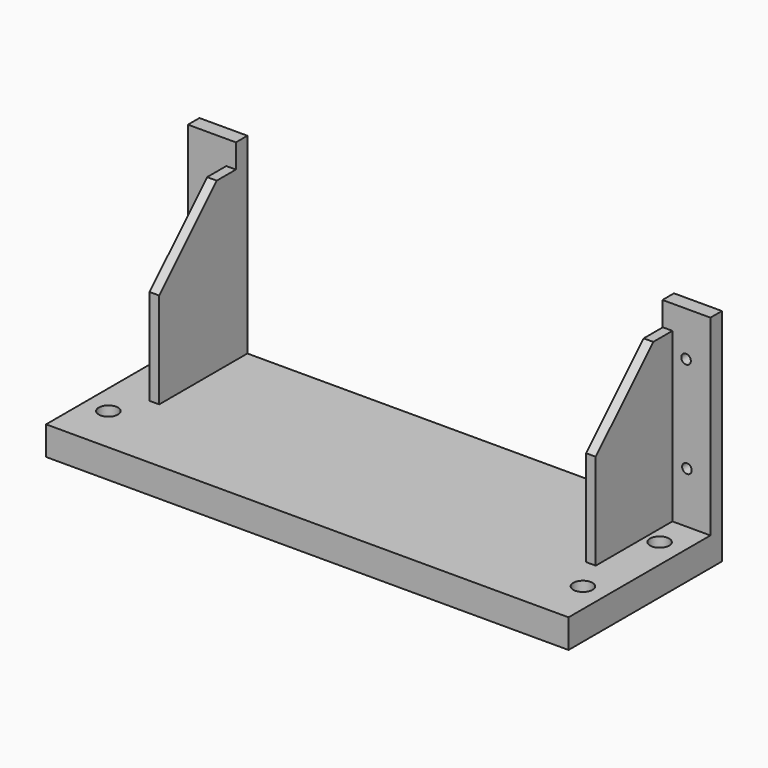
from build123d import *

# Parameters (mm, degrees)
F0_W     = 54.5
F0_H     = 20
F0_R     = 1
F1_DEPTH = 3
F2_W     = 5
F2_H     = 1.5
F3_DEPTH = 20
F4_W     = 1
F4_H     = 10
F5_DEPTH = 17.5
F6_SIZE  = 7.5
F8_D     = 1


# Not quite as in the source:
# - a feature names something its author has since deleted; it is built from what else it names


with BuildPart() as f1:
    # F0 (on Top) → F1 (new body)
    with BuildSketch(Plane.XY):
        Rectangle(F0_W, F0_H)
        with Locations((-24.75, -5)):
            Circle(F0_R, mode=Mode.SUBTRACT)
        with Locations((24.75, -5)):
            Circle(F0_R, mode=Mode.SUBTRACT)
        with Locations((-24.75, 5)):
            Circle(F0_R, mode=Mode.SUBTRACT)
        with Locations((24.75, 5)):
            Circle(F0_R, mode=Mode.SUBTRACT)
    extrude(amount=F1_DEPTH)

    # F2 (on face) → F3 (join)
    with BuildSketch(Plane.XY.offset(3)):
        with Locations((-24.75, 9.25)):
            Rectangle(F2_W, F2_H)
        with Locations((24.75, 9.25)):
            Rectangle(F2_W, F2_H)
    extrude(amount=F3_DEPTH)

    # F4 (on face) → F5 (join)
    with BuildSketch(Plane.XY.offset(3)):
        with Locations((-22.75, 3.5)):
            Rectangle(F4_W, F4_H)
        with Locations((22.7855359316, 3.5)):
            Rectangle(F4_W, F4_H)
    extrude(amount=F5_DEPTH)

    # F6
    f6_edges = [f1.edges().sort_by_distance(p)[0] for p in [
        (-22.75, -1.5, 20.5),
        (22.785536, -1.5, 20.5),
    ]]
    chamfer(f6_edges, length=F6_SIZE)

    # F8 (through all)
    with Locations(Plane(origin=(0, 10, 0), x_dir=(-1, 0, 0), z_dir=(0, 1, 0))):
        with Locations((24.8279795051, 8.3445450291), (24.7343406081, 18.3638688177), (-24.8004421592, 8.3445450291), (-24.7068032622, 18.3638688177)):
            Hole(F8_D / 2)


solid = f1.part
